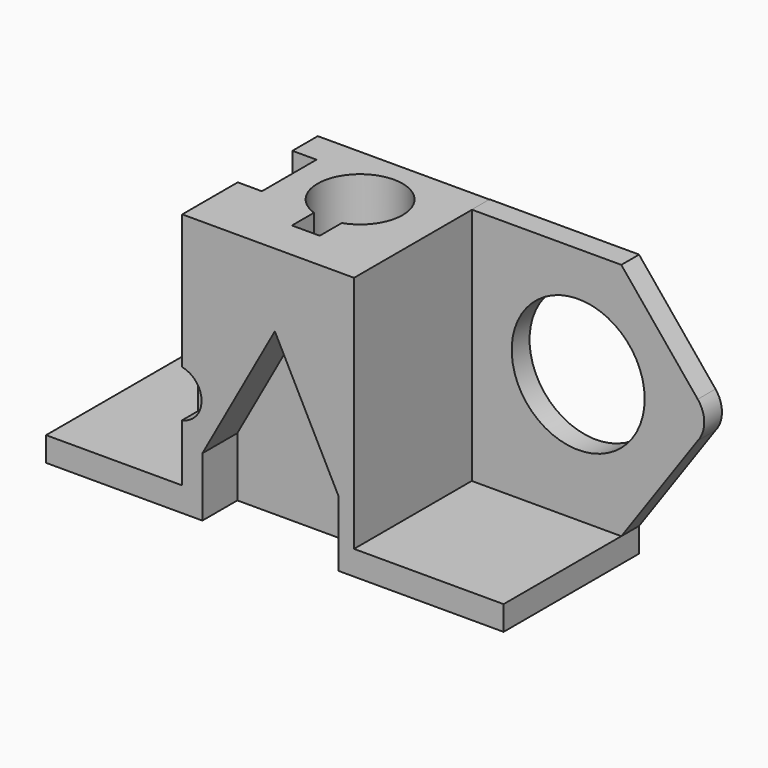
from build123d import *

# Parameters (mm, degrees)
F0_W      = 99.6
F0_H      = 27.37
F0_R      = 9.265
F1_DEPTH  = 5.32
F2_W      = 37.4
F2_H      = 27.37
F2_R      = 9.265
F3_DEPTH  = 51.95
F5_DEPTH  = 9.52
F7_DEPTH  = 22.25
F10_DEPTH = 37.475
F12_DEPTH = 7.5
F14_DEPTH = 5.25
F15_R     = 0.6044453377
F16_DEPTH = 25
F18_W     = 32.5579583809
F18_H     = 4.8552089012
F19_DEPTH = 52
F21_DEPTH = 4.825
F22_DEPTH = 25


with BuildPart() as f1:
    # F0 (on Top) → F1 (new body)
    with BuildSketch(Plane.XY):
        Rectangle(F0_W, F0_H)
        Circle(F0_R, mode=Mode.SUBTRACT)
    extrude(amount=F1_DEPTH)

    # F2 (on face) → F3 (join)
    with BuildSketch(Plane.XY.offset(5.32)):
        with Locations((-1.4579583809, 0)):
            Rectangle(F2_W, F2_H)
        Circle(F2_R, mode=Mode.SUBTRACT)
    extrude(amount=F3_DEPTH)

    # F4 (on face) → F5 (join)
    with BuildSketch(Plane.XZ.offset(13.685)):
        Polygon((-49.8, 0), (-15.7770887017, 0), (-15.7770887017, 12.8972763196), (0, 41.4250344038), (13.8749163598, 14.3025843427), (13.8749163598, 0), (49.8, 0), (49.8, 5.32), (17.2420416191, 5.32), (17.2420416191, 57.27), (-20.1579583809, 57.27), (-20.1579583809, 5.32), (-49.8, 5.32), align=None)
    extrude(amount=F5_DEPTH)

    # F6 (on face) → F7 (cut)
    with BuildSketch(Plane.XY.offset(57.27)):
        with BuildLine():
            ThreePointArc((3.0086552724, -8.7628887047), (-0.017033567, -9.264984342), (-3.0408557647, -8.7517667484))
            Line((-3.0408557647, -8.7517667484), (-3.0408557647, -14.7527681977))
            Line((-3.0408557647, -14.7527681977), (3.0086552724, -14.7527681977))
            Line((3.0086552724, -14.7527681977), (3.0086552724, -8.7628887047))
        make_face()
    extrude(amount=-F7_DEPTH, mode=Mode.SUBTRACT)

    # F9 (on face) → F10 (cut)
    with BuildSketch(Plane.XZ.offset(23.205)):
        with BuildLine():
            Line((-20.1579583809, 27.9725342989), (-20.1579583809, 17.8241562098))
            ThreePointArc((-20.1579583809, 17.8241562098), (-15.9551803728, 22.8983452544), (-20.1579583809, 27.9725342989))
        make_face()
    extrude(amount=-F10_DEPTH, mode=Mode.SUBTRACT)

    # F11 (on face) → F12 (join)
    with BuildSketch(Plane(origin=(-20.1579583809, 0, 0), x_dir=(0, -1, 0), z_dir=(-1, 0, 0))):
        Polygon((0, 17.7417956293), (0, 5.4170973599), (9.6006197855, 5.3354022093), (9.6006197855, 17.7417956293), align=None)
    extrude(amount=F12_DEPTH)

    # F13 (on face) → F14 (cut)
    with BuildSketch(Plane(origin=(-20.1579583809, 0, 0), x_dir=(0, -1, 0), z_dir=(-1, 0, 0))):
        Polygon((8.0970225025, 57.27), (-6.7709684372, 57.27), (-6.7709684372, 28.0677657574), (16.8139953166, 28.0677657574), (16.8139953166, 57.0610500872), align=None)
    extrude(amount=-F14_DEPTH, mode=Mode.SUBTRACT)

    # F15 (on face) → F16 (cut)
    with BuildSketch(Plane.XZ.offset(9.6006197855)):
        with Locations((-26.3735596091, 15.4167022556)):
            Circle(F15_R)
    extrude(amount=-F16_DEPTH, mode=Mode.SUBTRACT)

    # F18 (on face) → F19 (join)
    with BuildSketch(Plane.XY.offset(5.32)):
        with Locations((33.5210208096, 11.2573955494)):
            Rectangle(F18_W, F18_H)
    extrude(amount=F19_DEPTH)

    # F20 (on face) → F21 (join)
    with BuildSketch(Plane.XZ.offset(-8.8297910988)):
        with BuildLine():
            Line((49.8, 57.32), (49.8, 44.2806235084))
            ThreePointArc((49.8, 44.2806235084), (53.5530649007, 39.3313205539), (54.8859158534, 33.2646407187))
            ThreePointArc((54.8859158534, 33.2646407187), (53.5530649007, 27.1979608835), (49.8, 22.248657929))
            Line((49.8, 22.248657929), (49.8, 5.32))
            Line((49.8, 5.32), (66.4364546537, 29.0281493217))
            ThreePointArc((66.4364546537, 29.0281493217), (67.8548424387, 33.0029604957), (66.4364546537, 36.9777716696))
            Line((66.4364546537, 36.9777716696), (49.8, 57.32))
        make_face()
    extrude(amount=-F21_DEPTH)

    # F20 (on face) → F22 (cut)
    with BuildSketch(Plane.XZ.offset(-8.8297910988)):
        with BuildLine():
            ThreePointArc((25.9396215898, 33.2646407187), (40.4127687216, 18.7914935869), (54.8859158534, 33.2646407187))
            ThreePointArc((54.8859158534, 33.2646407187), (40.4127687216, 47.7377878505), (25.9396215898, 33.2646407187))
        make_face()
    extrude(amount=-F22_DEPTH, mode=Mode.SUBTRACT)


solid = f1.part
